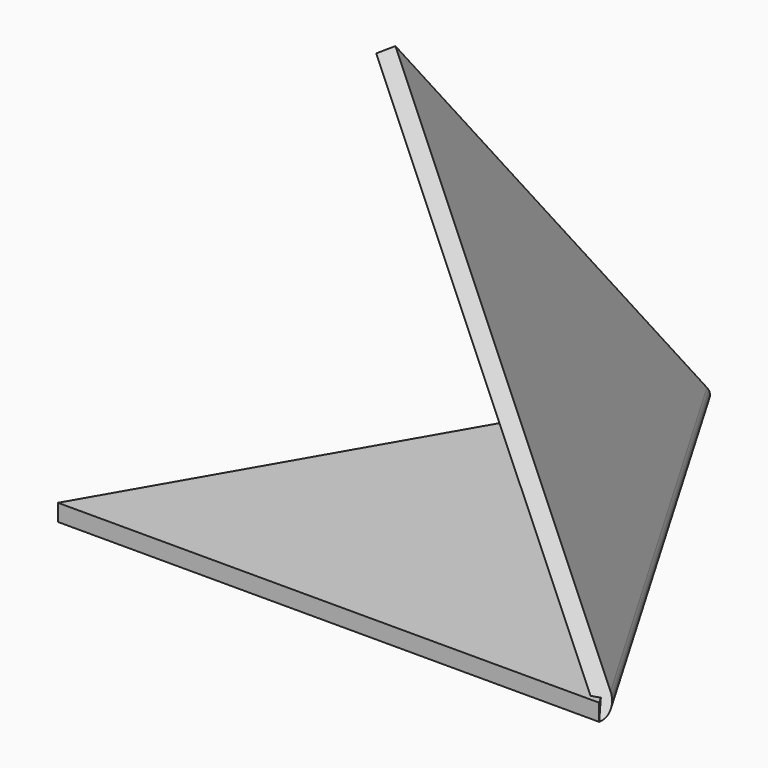
from build123d import *

# Parameters (mm, degrees)
F1_DEPTH    = 3.175
F5_DEPTH    = 3.175
F6_T1_DEPTH = 117.475


# Not quite as in the source:
# - a fillet or chamfer that OpenCascade refuses, or shapes differently, is made with other operations: its cross-section is extruded or revolved along the edge and cut away or added


with BuildPart() as f1:
    # F0 (on Top) → F1 (new body)
    with BuildSketch(Plane.XY):
        Polygon((50.8, 0), (0, 87.9881810245), (-50.8, 0), align=None)
    extrude(amount=F1_DEPTH)

    # F4 (on line) → F5 (join)
    with BuildSketch(Plane(origin=(30.2473107364, 17.7959839325, 17.4632910558), x_dir=(-0.3931673168, 0.8910065242, -0.226995231), z_dir=(0.7716343063, 0.4539904997, 0.445503225))):
        Polygon((6.5029600393, 75.2459340132), (-19.9755570322, -25.4006840255), (78.3980433443, 0), align=None)
    extrude(amount=F5_DEPTH)

    # F6: fillet of radius 3.175 on 1 edges, made by hand

    # F6_s2 → F6_t1 (cut)
    with BuildSketch(Plane(origin=(17.005719551, -29.012184774, 0.1101218851), x_dir=(-0.862716434, -0.5056880012, 0), z_dir=(-0.5056852899, 0.8627118085, -0.0032746052))):
        with BuildLine():
            ThreePointArc((-45.25402581, 4.1728704395), (-45.421662158, 1.7486197382), (-43.8259948462, -0.0841211704))
            Line((-43.8259948462, -0.0841211704), (-46.668506133, 1.3303591527))
            Line((-46.668506133, 1.3303591527), (-45.25402581, 4.1728704395))
        make_face()
    extrude(amount=F6_T1_DEPTH, mode=Mode.SUBTRACT)


solid = f1.part
